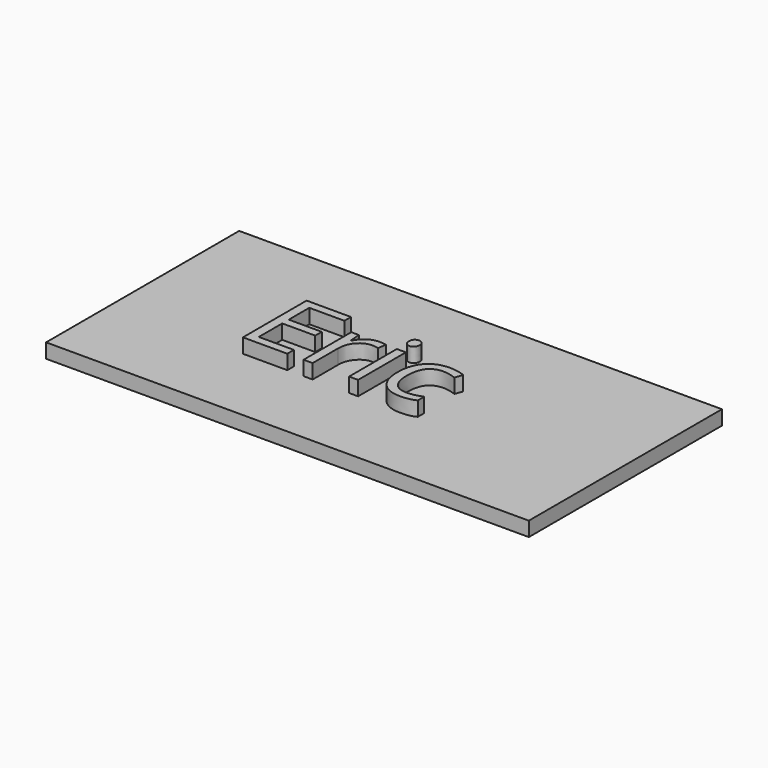
from build123d import *

# Parameters (mm, degrees)
F0_W         = 100
F0_H         = 50
F1_DEPTH     = 3
F2_TEXT_SIZE = 23.0925468107
F3_DEPTH     = 3


# Not quite as in the source:
# - Text() gives the source's letters only with a copy of the font that has no kerning and outlines rounded to 1/6400 em; it was checked with that copy


with BuildPart() as f1:
    # F0 (on Top) → F1 (new body)
    with BuildSketch(Plane.XY):
        with Locations((50, 25)):
            Rectangle(F0_W, F0_H)
    extrude(amount=F1_DEPTH)

    # F2 (on face) → F3 (join)
    with BuildSketch(Plane.XY.offset(3)):
        with Locations((25.1049865037, 16.7613886297)):
            Text('Eric', F2_TEXT_SIZE, font='Open Sans', text_align=(TextAlign.LEFT, TextAlign.BOTTOM))
    extrude(amount=F3_DEPTH)


solid = f1.part
